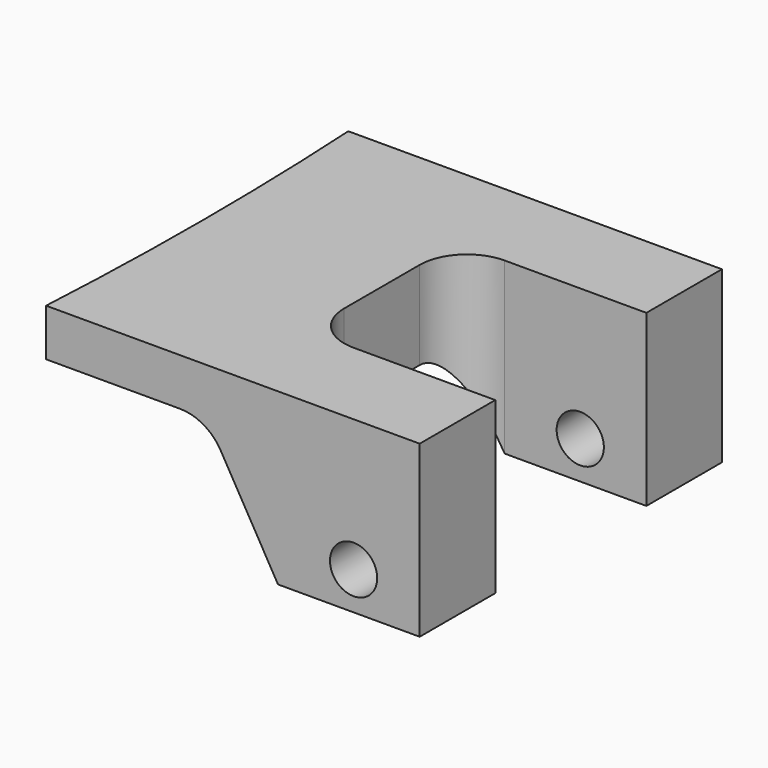
from build123d import *

# Parameters (mm, degrees)
F1_DEPTH      = 9
F1_DEPTH_BACK = 9
F3_DEPTH      = 25
F3_DEPTH_BACK = 25
F5_DEPTH      = 25
F5_DEPTH_BACK = 25
F6_R          = 2.5
F7_DEPTH      = 25
F7_DEPTH_BACK = 25


with BuildPart() as f1:
    # F0 (on Top) → F1 (new body, two sides)
    with BuildSketch(Plane.XY) as f1_sk:
        with BuildLine():
            ThreePointArc((-0.5590957934, 20), (-0.139801245, 10.0039065883), (0, 0))
            ThreePointArc((0, 0), (-0.139801245, -10.0039065883), (-0.5590957934, -20))
            Line((-0.5590957934, -20), (39, -20))
            Line((39, -20), (39, 20))
            Line((39, 20), (-0.5590957934, 20))
        make_face()
    extrude(amount=F1_DEPTH)
    extrude(f1_sk.sketch, amount=-F1_DEPTH_BACK)

    # F2 (on Front) → F3 (cut, two sides)
    with BuildSketch(Plane.XZ) as f3_sk:
        with BuildLine():
            Line((-2.6374068111, -9), (24, -9))
            Line((24, -9), (17.9378221735, 1.5))
            ThreePointArc((17.9378221735, 1.5), (16.1076951546, 3.3301270189), (13.6076951546, 4))
            Line((13.6076951546, 4), (-2.6374068111, 4))
            Line((-2.6374068111, 4), (-2.6374068111, -9))
        make_face()
    extrude(amount=-F3_DEPTH, mode=Mode.SUBTRACT)
    extrude(f3_sk.sketch, amount=F3_DEPTH_BACK, mode=Mode.SUBTRACT)

    # F4 (on Top) → F5 (cut, two sides)
    with BuildSketch(Plane.XY) as f5_sk:
        with BuildLine():
            ThreePointArc((19, -5), (20.4644660941, -8.5355339059), (24, -10))
            Line((24, -10), (41.5962561965, -10))
            Line((41.5962561965, -10), (41.5962561965, 10))
            Line((41.5962561965, 10), (24, 10))
            ThreePointArc((24, 10), (20.4644660941, 8.5355339059), (19, 5))
            Line((19, 5), (19, 0))
            Line((19, 0), (19, -5))
        make_face()
    extrude(amount=-F5_DEPTH, mode=Mode.SUBTRACT)
    extrude(f5_sk.sketch, amount=F5_DEPTH_BACK, mode=Mode.SUBTRACT)

    # F6 (on Front) → F7 (cut, two sides)
    with BuildSketch(Plane.XZ) as f7_sk:
        with Locations((32, -5)):
            Circle(F6_R)
    extrude(amount=-F7_DEPTH, mode=Mode.SUBTRACT)
    extrude(f7_sk.sketch, amount=F7_DEPTH_BACK, mode=Mode.SUBTRACT)


solid = f1.part
